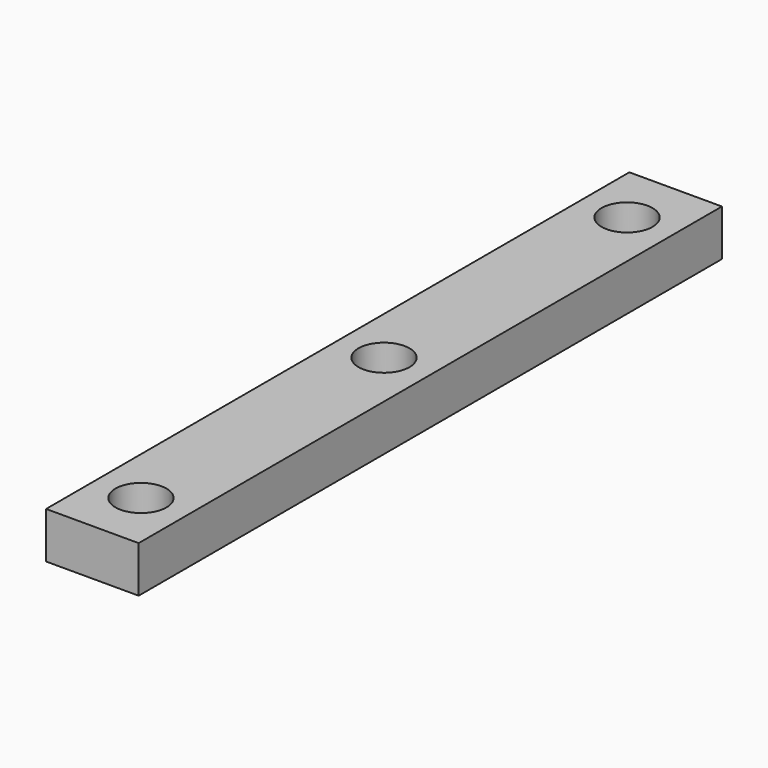
from build123d import *

# Parameters (mm, degrees)
F0_W     = 19.05
F0_H     = 150
F1_DEPTH = 9.525
F2_R     = 5.25
F3_DEPTH = 25.4
F4_R     = 5.25
F5_DEPTH = 25.4


# Not quite as in the source:
# - a length typed as a fraction of an inch, garbled in the dataset ("3 / 203.2 mm" for 3/8 in), is restored


with BuildPart() as f1:
    # F0 (on Top) → F1 (new body)
    with BuildSketch(Plane.XY):
        Rectangle(F0_W, F0_H)
    extrude(amount=F1_DEPTH)

    # F2 (on face) → F3 (cut)
    with BuildSketch(Plane.XY.offset(9.525)):
        with Locations((0, 62.5)):
            Circle(F2_R)
        with Locations((0, -62.5)):
            Circle(F2_R)
    extrude(amount=-F3_DEPTH, mode=Mode.SUBTRACT)

    # F4 (on face) → F5 (cut)
    with BuildSketch(Plane.XY.offset(9.525)):
        Circle(F4_R)
    extrude(amount=-F5_DEPTH, mode=Mode.SUBTRACT)


solid = f1.part
